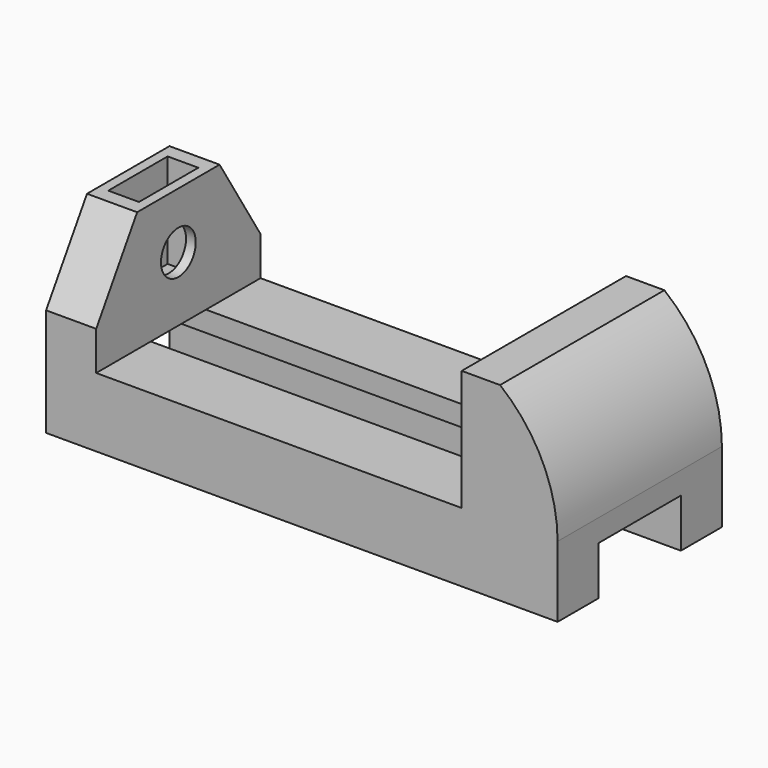
from build123d import *

# Parameters (mm, degrees)
F0_W       = 10
F0_H       = 3.305
F0_W_2     = 71.45
F0_W_3     = 8.75
F0_H_2     = 10.025
F0_W_4     = 9.8
F1_DEPTH   = 4
F2_DEPTH   = 13.5
F3_DEPTH   = 23.6
F4_SIZE2   = 10
F4_SIZE    = 16
F4_2_SIZE2 = 10
F4_2_SIZE  = 16
F6_DEPTH   = 40.151
F7_R       = 4.25
F8_DEPTH   = 25
F10_DEPTH  = 18.5


with BuildPart() as f1:
    # F0 (on Top) → F1 (new body)
    with BuildSketch(Plane.XY):
        with Locations((32.1862275445, -12.024865455)):
            Rectangle(F0_W, F0_H)
        with Locations((-17.2887724555, -12.024865455)):
            Rectangle(F0_W_2, F0_H)
        with Locations((22.8112275445, -12.024865455)):
            Rectangle(F0_W_3, F0_H)
        with Locations((22.8112275445, -18.689865455)):
            Rectangle(F0_W_3, F0_H_2)
        with Locations((32.1862275445, -18.689865455)):
            Rectangle(F0_W, F0_H_2)
        with Locations((-17.2887724555, -18.689865455)):
            Rectangle(F0_W_2, F0_H_2)
        with Locations((-57.9137724555, -18.689865455)):
            Rectangle(F0_W_4, F0_H_2)
        with Locations((-57.9137724555, -12.024865455)):
            Rectangle(F0_W_4, F0_H)
        with Locations((-57.9137724555, 4.770134545)):
            Rectangle(F0_W_4, F0_H)
        with Locations((-57.9137724555, 11.435134545)):
            Rectangle(F0_W_4, F0_H_2)
        with Locations((-17.2887724555, 11.435134545)):
            Rectangle(F0_W_2, F0_H_2)
        with Locations((-17.2887724555, 4.770134545)):
            Rectangle(F0_W_2, F0_H)
        with Locations((22.8112275445, 11.435134545)):
            Rectangle(F0_W_3, F0_H_2)
        with Locations((22.8112275445, 4.770134545)):
            Rectangle(F0_W_3, F0_H)
        with Locations((32.1862275445, 4.770134545)):
            Rectangle(F0_W, F0_H)
        with Locations((32.1862275445, 11.435134545)):
            Rectangle(F0_W, F0_H_2)
        Polygon((37.1862275445, 3.117634545), (27.1862275445, 3.117634545), (27.1862275445, -3.627365455), (27.1862275445, -10.372365455), (37.1862275445, -10.372365455), align=None)
    extrude(amount=-F1_DEPTH)

    # F0 (on Top) → F2 (join)
    with BuildSketch(Plane.XY):
        with Locations((-57.9137724555, -18.689865455)):
            Rectangle(F0_W_4, F0_H_2)
        with Locations((-17.2887724555, -18.689865455)):
            Rectangle(F0_W_2, F0_H_2)
        with Locations((22.8112275445, -18.689865455)):
            Rectangle(F0_W_3, F0_H_2)
        with Locations((32.1862275445, -18.689865455)):
            Rectangle(F0_W, F0_H_2)
        with Locations((32.1862275445, 11.435134545)):
            Rectangle(F0_W, F0_H_2)
        with Locations((22.8112275445, 11.435134545)):
            Rectangle(F0_W_3, F0_H_2)
        with Locations((-17.2887724555, 11.435134545)):
            Rectangle(F0_W_2, F0_H_2)
        with Locations((-57.9137724555, 11.435134545)):
            Rectangle(F0_W_4, F0_H_2)
    extrude(amount=-F2_DEPTH)

    # F0 (on Top) → F3 (join)
    with BuildSketch(Plane.XY):
        Polygon((-53.0137724555, 3.117634545), (-62.8137724555, 3.117634545), (-62.8137724555, -10.372365455), (-53.0137724555, -10.372365455), (-53.0137724555, -3.627365455), align=None)
        with Locations((-57.9137724555, -12.024865455)):
            Rectangle(F0_W_4, F0_H)
        with Locations((-57.9137724555, -18.689865455)):
            Rectangle(F0_W_4, F0_H_2)
        with Locations((-57.9137724555, 4.770134545)):
            Rectangle(F0_W_4, F0_H)
        with Locations((-57.9137724555, 11.435134545)):
            Rectangle(F0_W_4, F0_H_2)
        with Locations((32.1862275445, 11.435134545)):
            Rectangle(F0_W, F0_H_2)
        with Locations((22.8112275445, 4.770134545)):
            Rectangle(F0_W_3, F0_H)
        with Locations((22.8112275445, 11.435134545)):
            Rectangle(F0_W_3, F0_H_2)
        Polygon((27.1862275445, 3.117634545), (18.4362275445, 3.117634545), (18.4362275445, -3.627365455), (18.4362275445, -10.372365455), (27.1862275445, -10.372365455), (27.1862275445, -3.627365455), align=None)
        with Locations((22.8112275445, -18.689865455)):
            Rectangle(F0_W_3, F0_H_2)
        with Locations((22.8112275445, -12.024865455)):
            Rectangle(F0_W_3, F0_H)
        with Locations((32.1862275445, -18.689865455)):
            Rectangle(F0_W, F0_H_2)
        with Locations((32.1862275445, -12.024865455)):
            Rectangle(F0_W, F0_H)
        Polygon((37.1862275445, 3.117634545), (27.1862275445, 3.117634545), (27.1862275445, -3.627365455), (27.1862275445, -10.372365455), (37.1862275445, -10.372365455), align=None)
        with Locations((32.1862275445, 4.770134545)):
            Rectangle(F0_W, F0_H)
    extrude(amount=F3_DEPTH)

    # F4
    f4_edges = [f1.edges().sort_by_distance(p)[0] for p in [
        (-57.913772, 16.447635, 23.6),
    ]]
    f4_side = f1.faces().sort_by_distance((-9.085188, 16.447635, -0.574122))[0]
    chamfer(f4_edges, length=F4_SIZE, length2=F4_SIZE2, reference=f4_side)

    # F4#2
    f4_2_edges = [f1.edges().sort_by_distance(p)[0] for p in [
        (-57.913772, -23.702365, 23.6),
    ]]
    f4_2_side = f1.faces().sort_by_distance((-9.085188, -23.702365, -0.574122))[0]
    chamfer(f4_2_edges, length=F4_2_SIZE, length2=F4_2_SIZE2, reference=f4_2_side)

    # F5 (on face) → F6 (cut, through all)
    with BuildSketch(Plane(origin=(0, 16.447634545, 0), x_dir=(-1, 0, 0), z_dir=(0, 1, 0))):
        with BuildLine():
            ThreePointArc((-37.1862275445, 0.3616424249), (-34.1889830456, 13.252952829), (-25.9362275445, 23.6))
            Line((-25.9362275445, 23.6), (-37.1862275445, 23.6))
            Line((-37.1862275445, 23.6), (-37.1862275445, 0.3616424249))
        make_face()
    extrude(amount=-F6_DEPTH, mode=Mode.SUBTRACT)

    # F7 (on face) → F8 (cut)
    with BuildSketch(Plane(origin=(-62.8137724555, 0, 0), x_dir=(0, -1, 0), z_dir=(-1, 0, 0))):
        with Locations((3.627365455, 12.6)):
            Circle(F7_R)
    extrude(amount=-F8_DEPTH, mode=Mode.SUBTRACT)

    # F9 (on face) → F10 (cut)
    with BuildSketch(Plane.XY.offset(23.6)):
        Polygon((-54.9137724555, -10.877365455), (-54.9137724555, -3.627365455), (-54.9137724555, 3.622634545), (-57.9137724555, 3.622634545), (-60.9137724555, 3.622634545), (-60.9137724555, -3.627365455), (-60.9137724555, -10.877365455), (-57.9137724555, -10.877365455), align=None)
    extrude(amount=-F10_DEPTH, mode=Mode.SUBTRACT)


solid = f1.part
